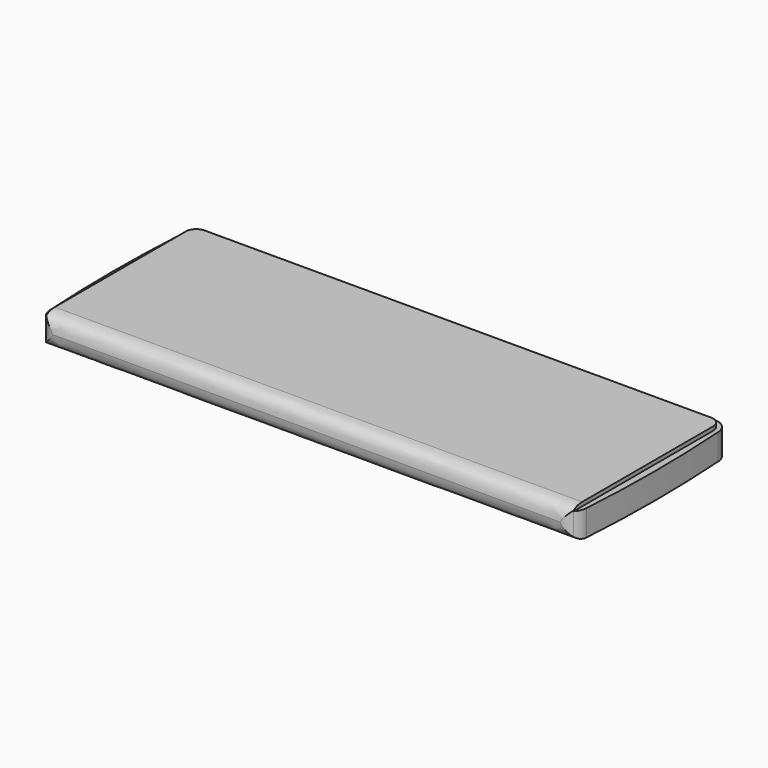
from build123d import *

# Parameters (mm, degrees)
F1_DEPTH    = 25.4
F2_DEPTH    = 22.098
F3_T1_DEPTH = 495.3


# Not quite as in the source:
# - a fillet or chamfer that OpenCascade refuses, or shapes differently, is made with other operations: its cross-section is extruded or revolved along the edge and cut away or added


with BuildPart() as f1:
    # F0 (on Top) → F1 (new body)
    with BuildSketch(Plane.XY):
        with BuildLine():
            ThreePointArc((215.9, -82.55), (220.7013488144, -81.6074252948), (224.79, -78.9196141042))
            Line((224.79, -78.9196141042), (224.79, -69.85))
            Line((224.79, -69.85), (224.79, 69.85))
            ThreePointArc((224.79, 69.85), (222.1861792847, 76.1361792847), (215.9, 78.74))
            Line((215.9, 78.74), (-215.9, 78.74))
            ThreePointArc((-215.9, 78.74), (-222.1861792847, 76.1361792847), (-224.79, 69.85))
            Line((-224.79, 69.85), (-224.79, -69.85))
            Line((-224.79, -69.85), (-224.79, -78.9196141042))
            ThreePointArc((-224.79, -78.9196141042), (-220.7013488144, -81.6074252948), (-215.9, -82.55))
            Line((-215.9, -82.55), (215.9, -82.55))
        make_face()
    extrude(amount=F1_DEPTH)

    # F0 (on Top) → F2 (join)
    with BuildSketch(Plane.XY):
        with BuildLine():
            ThreePointArc((228.6, 69.85), (224.8802561211, 78.8302561211), (215.9, 82.55))
            Line((215.9, 82.55), (-215.9, 82.55))
            ThreePointArc((-215.9, 82.55), (-224.8802561211, 78.8302561211), (-228.6, 69.85))
            ThreePointArc((-228.6, 69.85), (-230.7318859092, 0), (-228.6, -69.85))
            ThreePointArc((-228.6, -69.85), (-227.6088214608, -74.7686888497), (-224.79, -78.9196141042))
            Line((-224.79, -78.9196141042), (-224.79, -69.85))
            Line((-224.79, -69.85), (-224.79, 69.85))
            ThreePointArc((-224.79, 69.85), (-222.1861792847, 76.1361792847), (-215.9, 78.74))
            Line((-215.9, 78.74), (215.9, 78.74))
            ThreePointArc((215.9, 78.74), (222.1861792847, 76.1361792847), (224.79, 69.85))
            Line((224.79, 69.85), (224.79, -69.85))
            Line((224.79, -69.85), (224.79, -78.9196141042))
            ThreePointArc((224.79, -78.9196141042), (227.6088214608, -74.7686888497), (228.6, -69.85))
            ThreePointArc((228.6, -69.85), (230.9555402084, 0), (228.6, 69.85))
        make_face()
    extrude(amount=F2_DEPTH)

    # F3: fillet of radius 12.7 on 4 edges, made by hand

    # F3_s2 → F3_t1 (cut)
    with BuildSketch(Plane.YZ.offset(-247.65)):
        with BuildLine():
            add(Edge.make_bspline(
                [(-69.85, 0), (-82.55, 0), (-82.55, 12.7)],
                knots=[0, 0, 0, 1, 1, 1], degree=2, weights=[1, 1, 1]))
            Line((-82.55, 12.7), (-82.55, 0))
            Line((-82.55, 0), (-69.85, 0))
        make_face()
        with BuildLine():
            add(Edge.make_bspline(
                [(-69.85, 25.4), (-82.55, 25.4), (-82.55, 12.7)],
                knots=[0, 0, 0, 1, 1, 1], degree=2, weights=[1, 1, 1]))
            Line((-82.55, 12.7), (-82.55, 25.4))
            Line((-82.55, 25.4), (-69.85, 25.4))
        make_face()
    extrude(amount=F3_T1_DEPTH, mode=Mode.SUBTRACT)


solid = f1.part
